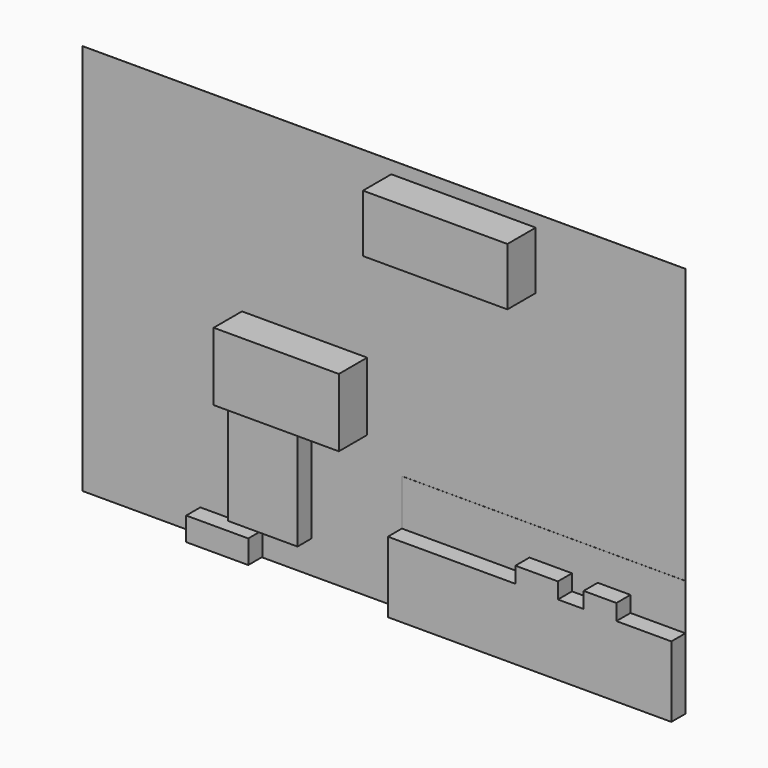
from build123d import *

# Parameters (mm, degrees)
F1_DEPTH = 4000
F0_W     = 16300
F0_H     = 6500
F2_DEPTH = 15
F0_W_2   = 7003.8146972656
F0_H_2   = 2644.2041069269
F3_DEPTH = 5
F4_DEPTH = 15
F0_W_3   = 4800
F0_H_3   = 1800
F0_W_4   = 3700
F0_W_5   = 7860.5866823946
F0_H_4   = 12313.6479878812
F5_DEPTH = 2000


with BuildPart() as f1:
    # F0 (on Front) → F1 (new body)
    with BuildSketch(Plane.XZ):
        Polygon((32126.2728316861, 23700), (18000, 23700), (18000, 16013.6479878812), (25860.5866823946, 16013.6479878812), (32126.2728316861, 16013.6479878812), align=None)
    extrude(amount=F1_DEPTH)


with BuildPart() as f1b:
    # F0 (on Front) → F1, piece 2 (new body)
    with BuildSketch(Plane.XZ):
        with Locations((43000, 39550)):
            Rectangle(F0_W, F0_H)
    extrude(amount=F1_DEPTH)


with BuildPart() as f2:
    # F0 (on Front) → F2 (new body)
    with BuildSketch(Plane.XZ):
        Polygon((36055.7479858398, 13200), (36055.7479858398, 8000), (50450, 8000), (50450, 9800), (55250, 9800), (55250, 8000), (58150, 8000), (58150, 9800), (61850, 9800), (61850, 8000), (68050, 8000), (68050, 13200), align=None)
    extrude(amount=F2_DEPTH)


with BuildPart() as f3:
    # F0 (on Front) → F3 (new body)
    with BuildSketch(Plane.XZ):
        Polygon((0, 44200), (0, 0), (35650, 0), (36055.7479858399, 0), (36055.7479858399, 8000), (36055.7479858398, 13200), (68050, 13200), (68050, 44200), align=None)
        with Locations((16801.9073486328, 1377.8979465365)):
            Rectangle(F0_W_2, F0_H_2, mode=Mode.SUBTRACT)
        Polygon((18000, 16013.6479878812), (18000, 23700), (32126.2728316861, 23700), (32126.2728316861, 16013.6479878812), (25860.5866823946, 16013.6479878812), (25860.5866823946, 3700), (18000, 3700), align=None, mode=Mode.SUBTRACT)
        with Locations((43000, 39550)):
            Rectangle(F0_W, F0_H, mode=Mode.SUBTRACT)
    extrude(amount=F3_DEPTH)

    # F0 (on Front) → F4 (join)
    with BuildSketch(Plane.XZ):
        Polygon((36055.7479858398, 13200), (36055.7479858398, 8000), (50450, 8000), (50450, 9800), (55250, 9800), (55250, 8000), (58150, 8000), (58150, 9800), (61850, 9800), (61850, 8000), (68050, 8000), (68050, 13200), align=None)
    extrude(amount=F4_DEPTH)

    # F0 (on Front) → F5 (join)
    with BuildSketch(Plane.XZ):
        Polygon((36055.7479858399, 8000), (36055.7479858399, 0), (68050, 0), (68050, 8000), (61850, 8000), (58150, 8000), (55250, 8000), (50450, 8000), align=None)
        with Locations((52850, 8900)):
            Rectangle(F0_W_3, F0_H_3)
        with Locations((60000, 8900)):
            Rectangle(F0_W_4, F0_H_3)
        with Locations((21930.2933411973, 9856.8239939406)):
            Rectangle(F0_W_5, F0_H_4)
        with Locations((16801.9073486328, 1377.8979465365)):
            Rectangle(F0_W_2, F0_H_2)
    extrude(amount=F5_DEPTH)


solid = Compound([f1.part, f1b.part, f2.part, f3.part])
